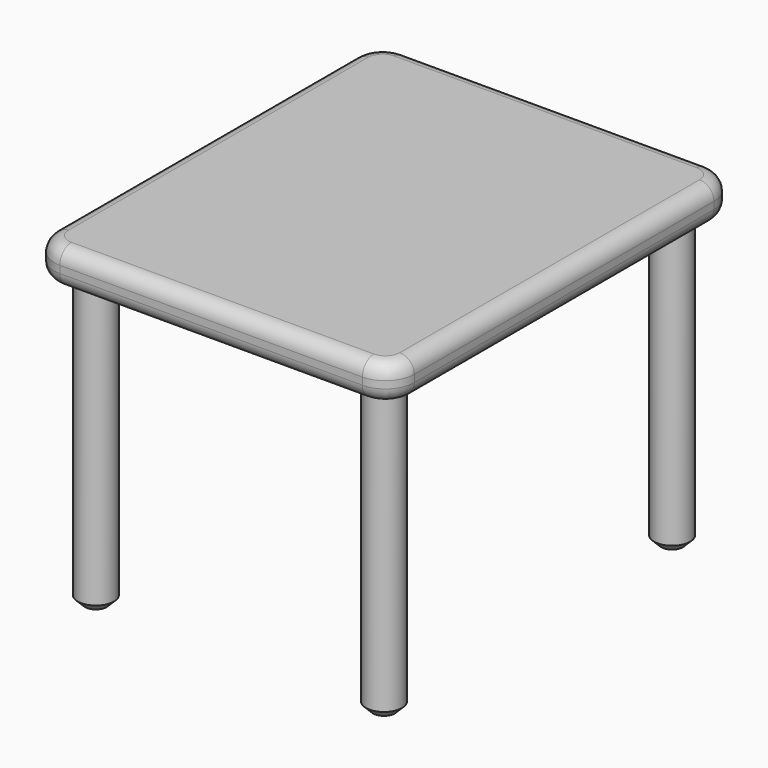
from build123d import *

# Parameters (mm, degrees)
F0_W          = 127
F0_H          = 152.4
F1_DEPTH      = 12.7
F2_T          = -5.08
F3_R          = 6.35
F4_DEPTH      = 101.6
F4_DEPTH_BACK = 7.62
F5_R          = 10.16
F6_T1_DEPTH   = 132.08
F6_T3_DEPTH   = 106.68
F6_T6_ANGLE   = 90
F6_T8_ANGLE   = 90
F6_T10_ANGLE  = 90
F6_T12_ANGLE  = 90
F6_T14_ANGLE  = 90
F6_T16_ANGLE  = 90
F6_T18_ANGLE  = 90
F6_T20_ANGLE  = 90
F7_SIZE       = 2.54


# Not quite as in the source:
# - a fillet or chamfer that OpenCascade refuses, or shapes differently, is made with other operations: its cross-section is extruded or revolved along the edge and cut away or added


with BuildPart() as f1:
    # F0 (on Top) → F1 (new body)
    with BuildSketch(Plane.XY):
        Rectangle(F0_W, F0_H)
    extrude(amount=-F1_DEPTH)

    # F2
    f2_openings = [f1.faces().sort_by_distance(p)[0] for p in [
        (0, 0, -12.7),
    ]]
    offset(amount=F2_T, openings=f2_openings)

    # F3 (on face) → F4 (join, two sides)
    with BuildSketch(Plane(origin=(0, 0, -12.7), x_dir=(1, 0, 0), z_dir=(0, 0, -1))) as f4_sk:
        with Locations((-50.8, 63.5)):
            Circle(F3_R)
        with Locations((50.8, 63.5)):
            Circle(F3_R)
        with Locations((50.8, -63.5)):
            Circle(F3_R)
        with Locations((-50.8, -63.5)):
            Circle(F3_R)
    extrude(amount=F4_DEPTH)
    extrude(f4_sk.sketch, amount=-F4_DEPTH_BACK)

    # F5
    f5_edges = [f1.edges().sort_by_distance(p)[0] for p in [
        (-63.5, -76.2, -6.35),
        (-63.5, 76.2, -6.35),
        (63.5, 76.2, -6.35),
        (63.5, -76.2, -6.35),
    ]]
    fillet(f5_edges, radius=F5_R)

    # F6: fillet of radius 5.08 on 18 edges, made by hand

    # F6_s2 → F6_t1 (cut)
    with BuildSketch(Plane.XZ.offset(-66.04)):
        with BuildLine():
            ThreePointArc((-58.42, 0), (-62.0121024484, -1.4878975516), (-63.5, -5.08))
            Line((-63.5, -5.08), (-63.5, 0))
            Line((-63.5, 0), (-58.42, 0))
        make_face()
        with BuildLine():
            ThreePointArc((-58.42, -12.7), (-62.0121024484, -11.2121024484), (-63.5, -7.62))
            Line((-63.5, -7.62), (-63.5, -12.7))
            Line((-63.5, -12.7), (-58.42, -12.7))
        make_face()
        with BuildLine():
            ThreePointArc((58.42, 0), (62.0121024484, -1.4878975516), (63.5, -5.08))
            Line((63.5, -5.08), (63.5, 0))
            Line((63.5, 0), (58.42, 0))
        make_face()
        with BuildLine():
            ThreePointArc((58.42, -12.7), (62.0121024484, -11.2121024484), (63.5, -7.62))
            Line((63.5, -7.62), (63.5, -12.7))
            Line((63.5, -12.7), (58.42, -12.7))
        make_face()
    extrude(amount=F6_T1_DEPTH, mode=Mode.SUBTRACT)

    # F6_s4 → F6_t3 (cut)
    with BuildSketch(Plane.YZ.offset(-53.34)):
        with BuildLine():
            ThreePointArc((-76.2, -5.08), (-74.7121024484, -1.4878975516), (-71.12, 0))
            Line((-71.12, 0), (-76.2, 0))
            Line((-76.2, 0), (-76.2, -5.08))
        make_face()
        with BuildLine():
            ThreePointArc((-76.2, -7.62), (-74.7121024484, -11.2121024484), (-71.12, -12.7))
            Line((-71.12, -12.7), (-76.2, -12.7))
            Line((-76.2, -12.7), (-76.2, -7.62))
        make_face()
        with BuildLine():
            ThreePointArc((71.12, 0), (74.7121024484, -1.4878975516), (76.2, -5.08))
            Line((76.2, -5.08), (76.2, 0))
            Line((76.2, 0), (71.12, 0))
        make_face()
        with BuildLine():
            ThreePointArc((71.12, -12.7), (74.7121024484, -11.2121024484), (76.2, -7.62))
            Line((76.2, -7.62), (76.2, -12.7))
            Line((76.2, -12.7), (71.12, -12.7))
        make_face()
    extrude(amount=F6_T3_DEPTH, mode=Mode.SUBTRACT)

    # F6_s5 → F6_t6 (revolve, cut)
    with BuildSketch(Plane.YZ.offset(-53.34)):
        with BuildLine():
            ThreePointArc((-71.12, 0), (-74.7121024484, -1.4878975516), (-76.2, -5.08))
            Line((-76.2, -5.08), (-76.2, 0))
            Line((-76.2, 0), (-71.12, 0))
        make_face()
    revolve(axis=Axis((-53.34, -66.04, 0), (0, 0, -1)), revolution_arc=F6_T6_ANGLE, mode=Mode.SUBTRACT)

    # F6_s7 → F6_t8 (revolve, cut)
    with BuildSketch(Plane.YZ.offset(53.34)):
        with BuildLine():
            ThreePointArc((-71.12, 0), (-74.7121024484, -1.4878975516), (-76.2, -5.08))
            Line((-76.2, -5.08), (-76.2, 0))
            Line((-76.2, 0), (-71.12, 0))
        make_face()
    revolve(axis=Axis((53.34, -66.04, 0), (0, 0, 1)), revolution_arc=F6_T8_ANGLE, mode=Mode.SUBTRACT)

    # F6_s9 → F6_t10 (revolve, cut)
    with BuildSketch(Plane.YZ.offset(-53.34)):
        with BuildLine():
            ThreePointArc((71.12, 0), (74.7121024484, -1.4878975516), (76.2, -5.08))
            Line((76.2, -5.08), (76.2, 0))
            Line((76.2, 0), (71.12, 0))
        make_face()
    revolve(axis=Axis((-53.34, 66.04, 0), (0, 0, 1)), revolution_arc=F6_T10_ANGLE, mode=Mode.SUBTRACT)

    # F6_s11 → F6_t12 (revolve, cut)
    with BuildSketch(Plane.YZ.offset(53.34)):
        with BuildLine():
            ThreePointArc((71.12, 0), (74.7121024484, -1.4878975516), (76.2, -5.08))
            Line((76.2, -5.08), (76.2, 0))
            Line((76.2, 0), (71.12, 0))
        make_face()
    revolve(axis=Axis((53.34, 66.04, 0), (0, 0, -1)), revolution_arc=F6_T12_ANGLE, mode=Mode.SUBTRACT)

    # F6_s13 → F6_t14 (revolve, cut)
    with BuildSketch(Plane.YZ.offset(-53.34)):
        with BuildLine():
            ThreePointArc((-76.2, -7.62), (-74.7121024484, -11.2121024484), (-71.12, -12.7))
            Line((-71.12, -12.7), (-76.2, -12.7))
            Line((-76.2, -12.7), (-76.2, -7.62))
        make_face()
    revolve(axis=Axis((-53.34, -66.04, -12.7), (0, 0, -1)), revolution_arc=F6_T14_ANGLE, mode=Mode.SUBTRACT)

    # F6_s15 → F6_t16 (revolve, cut)
    with BuildSketch(Plane.YZ.offset(53.34)):
        with BuildLine():
            ThreePointArc((-76.2, -7.62), (-74.7121024484, -11.2121024484), (-71.12, -12.7))
            Line((-71.12, -12.7), (-76.2, -12.7))
            Line((-76.2, -12.7), (-76.2, -7.62))
        make_face()
    revolve(axis=Axis((53.34, -66.04, -12.7), (0, 0, 1)), revolution_arc=F6_T16_ANGLE, mode=Mode.SUBTRACT)

    # F6_s17 → F6_t18 (revolve, cut)
    with BuildSketch(Plane.YZ.offset(-53.34)):
        with BuildLine():
            ThreePointArc((71.12, -12.7), (74.7121024484, -11.2121024484), (76.2, -7.62))
            Line((76.2, -7.62), (76.2, -12.7))
            Line((76.2, -12.7), (71.12, -12.7))
        make_face()
    revolve(axis=Axis((-53.34, 66.04, -12.7), (0, 0, 1)), revolution_arc=F6_T18_ANGLE, mode=Mode.SUBTRACT)

    # F6_s19 → F6_t20 (revolve, cut)
    with BuildSketch(Plane.YZ.offset(53.34)):
        with BuildLine():
            ThreePointArc((71.12, -12.7), (74.7121024484, -11.2121024484), (76.2, -7.62))
            Line((76.2, -7.62), (76.2, -12.7))
            Line((76.2, -12.7), (71.12, -12.7))
        make_face()
    revolve(axis=Axis((53.34, 66.04, -12.7), (0, 0, -1)), revolution_arc=F6_T20_ANGLE, mode=Mode.SUBTRACT)

    # F7
    f7_edges = [f1.edges().sort_by_distance(p)[0] for p in [
        (-57.15, -63.5, -114.3),
        (44.45, -63.5, -114.3),
        (-57.15, 63.5, -114.3),
        (44.45, 63.5, -114.3),
    ]]
    chamfer(f7_edges, length=F7_SIZE)


solid = f1.part
